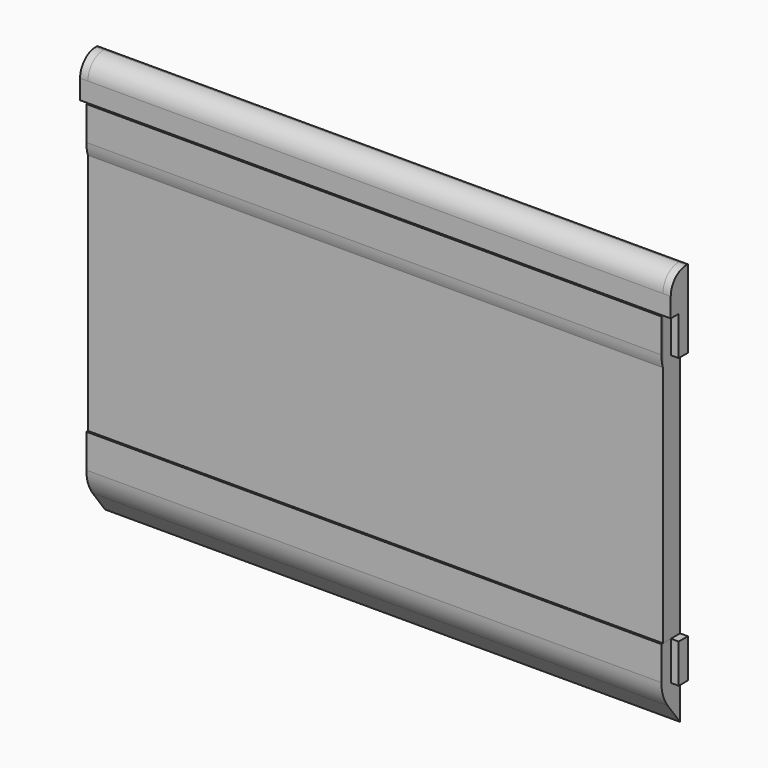
from build123d import *

# Parameters (mm, degrees)
F1_DEPTH  = 147.5
F2_R      = 10
F2_2_R    = 10
F4_DEPTH  = 147.5
F5_W      = 2.95
F5_H      = 10
F6_DEPTH  = 2
F7_W      = 2.95
F7_H      = 10
F8_DEPTH  = 2
F9_R      = 5
F11_DEPTH = 2
F13_DEPTH = 2


with BuildPart() as f1:
    # F0 (on Right) → F1 (new body)
    with BuildSketch(Plane.YZ):
        Polygon((35.9455486238, 28.1918546259), (35.9455486238, 38.1918546259), (32.9455486238, 38.1918546259), (32.9455486238, 48.1918546259), (29.9455486238, 48.1918546259), (29.9455486238, 36.1918546259), align=None)
    extrude(amount=F1_DEPTH)

    # F2
    f2_edges = [f1.edges().sort_by_distance(p)[0] for p in [
        (73.75, 29.945549, 36.191855),
    ]]
    fillet(f2_edges, radius=F2_R)


with BuildPart() as f1b:
    # F0 (on Right) → F1, piece 2 (new body)
    with BuildSketch(Plane.YZ):
        Polygon((35.9455486238, -45.8081453741), (35.9455486238, -35.8081453741), (32.9455486238, -35.8081453741), (32.9455486238, -25.8081453741), (29.9455486238, -25.8081453741), (29.9455486238, -37.8081453741), align=None)
    extrude(amount=F1_DEPTH)

    # F2#2
    f2_2_edges = [f1b.edges().sort_by_distance(p)[0] for p in [
        (73.75, 29.945549, -37.808145),
    ]]
    fillet(f2_2_edges, radius=F2_2_R)


with BuildPart() as f4:
    # F3 (on face) → F4 (new body)
    with BuildSketch(Plane(origin=(0, 0, 0), x_dir=(0, -1, 0), z_dir=(-1, 0, 0))):
        Polygon((-30.4455486238, 58.1918546259), (-35.9455486238, 58.1918546259), (-35.9455486238, -35.8081453741), (-32.9455486238, -35.8081453741), (-32.9455486238, -25.8081453741), (-30.4455486238, -25.8081453741), align=None)
    extrude(amount=-F4_DEPTH)

    # F5 (on face) → F6 (join)
    with BuildSketch(Plane(origin=(0, 0, 0), x_dir=(0, -1, 0), z_dir=(-1, 0, 0))):
        with Locations((-34.4705486238, 43.1918546259)):
            Rectangle(F5_W, F5_H)
        with Locations((-34.4705486238, -30.8081453741)):
            Rectangle(F5_W, F5_H)
    extrude(amount=F6_DEPTH)

    # F7 (on face) → F8 (join)
    with BuildSketch(Plane.YZ.offset(147.5)):
        with Locations((34.4705486238, 43.1918546259)):
            Rectangle(F7_W, F7_H)
        with Locations((34.4705486238, -30.8081453741)):
            Rectangle(F7_W, F7_H)
    extrude(amount=F8_DEPTH)

    # F9
    f9_edges = [f4.edges().sort_by_distance(p)[0] for p in [
        (73.75, 30.445549, 58.191855),
    ]]
    fillet(f9_edges, radius=F9_R)

    # F10 (on face) → F11 (join)
    with BuildSketch(Plane(origin=(0, 0, 0), x_dir=(0, -1, 0), z_dir=(-1, 0, 0))):
        with BuildLine():
            Line((-35.9455486238, 48.1918546259), (-32.9955486238, 48.1918546259))
            Line((-32.9955486238, 48.1918546259), (-30.4455486238, 48.1918546259))
            Line((-30.4455486238, 48.1918546259), (-30.4455486238, 53.1918546259))
            ThreePointArc((-30.4455486238, 53.1918546259), (-31.9100147179, 56.7273885319), (-35.4455486238, 58.1918546259))
            Line((-35.4455486238, 58.1918546259), (-35.9455486238, 58.1918546259))
            Line((-35.9455486238, 58.1918546259), (-35.9455486238, 48.1918546259))
        make_face()
    extrude(amount=F11_DEPTH)

    # F12 (on face) → F13 (join)
    with BuildSketch(Plane.YZ.offset(147.5)):
        with BuildLine():
            Line((30.4455486238, 48.1918546259), (32.9955486238, 48.1918546259))
            Line((32.9955486238, 48.1918546259), (35.9455486238, 48.1918546259))
            Line((35.9455486238, 48.1918546259), (35.9455486238, 58.1918546259))
            Line((35.9455486238, 58.1918546259), (35.4455486238, 58.1918546259))
            ThreePointArc((35.4455486238, 58.1918546259), (31.9100147179, 56.7273885319), (30.4455486238, 53.1918546259))
            Line((30.4455486238, 53.1918546259), (30.4455486238, 48.1918546259))
        make_face()
    extrude(amount=F13_DEPTH)


solid = Compound([f1.part, f1b.part, f4.part])
